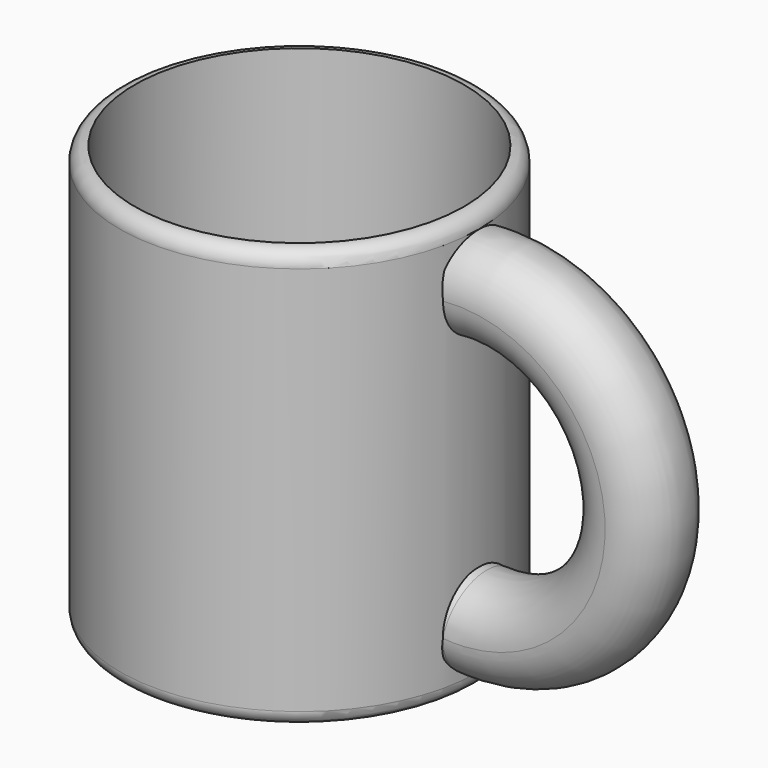
from build123d import *

# Parameters (mm, degrees)
F0_R     = 38.1
F1_DEPTH = 88.9
F2_T     = -3.175
F4_R     = 9.525
F7_R     = 3.17499


# Not quite as in the source:
# - a fillet or chamfer is up to 0.001 mm smaller than in the source, because OpenCascade refuses the exact size


with BuildPart() as f1:
    # F0 (on Top) → F1 (new body)
    with BuildSketch(Plane.XY):
        Circle(F0_R)
    extrude(amount=F1_DEPTH)

    # F2
    f2_openings = [f1.faces().sort_by_distance(p)[0] for p in [
        (0, 0, 88.9),
    ]]
    offset(amount=F2_T, openings=f2_openings)

    # F6: sweep along a path in F5
    with BuildLine(Plane.XZ) as f6_path:
        ThreePointArc((38.00738, 13.075479), (72.566927, 44.674488), (38.060052, 76.331008))
    # F4 (on offset) → F6 (sweep)
    with BuildSketch(Plane.YZ.offset(38.1)):
        with Locations((0, 76.129749)):
            Circle(F4_R)
        with Locations((0, 13.206737)):
            Circle(F4_R)
    sweep(path=f6_path.line)

    # F7 (radius 3.175 in the source; OpenCascade refuses exactly that, so slightly less here)
    f7_edges = [f1.edges().sort_by_distance(p)[0] for p in [
        (-38.1, 0, 88.9),
        (-38.1, 0, 0),
    ]]
    fillet(f7_edges, radius=F7_R)


solid = f1.part
